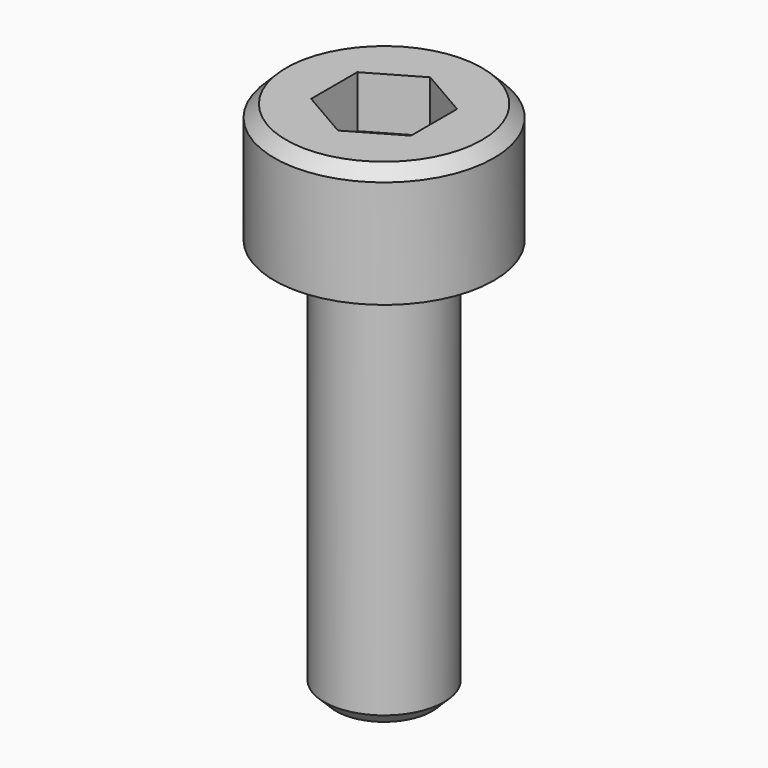
from build123d import *

# Parameters (mm, degrees)
F2_R      = 1.5
F3_DEPTH  = 10
F2_R_2    = 2.75
F3_FACE_R = 1.5
F4_DEPTH  = 3
F5_SIZE   = 0.3
F7_DEPTH  = 1.3


with BuildPart() as f3:
    # F2 (on Top) → F3 (new body)
    with BuildSketch(Plane.XY):
        Circle(F2_R)
    extrude(amount=-F3_DEPTH)

    # F2 (on Top) + F3_face (on face) → F4 (join)
    with BuildSketch(Plane.XY):
        Circle(F2_R_2)
        Circle(F2_R, mode=Mode.SUBTRACT)
    with BuildSketch(Plane.XY):
        Circle(F3_FACE_R)
    extrude(amount=F4_DEPTH)

    # F5
    f5_edges = [f3.edges().sort_by_distance(p)[0] for p in [
        (-1.5, 0, -10),
        (-2.75, 0, 3),
    ]]
    chamfer(f5_edges, length=F5_SIZE)

    # F6 (on face) → F7 (cut)
    with BuildSketch(Plane.XY.offset(3)):
        Polygon((1.25, -0.7216878365), (1.25, 0.7216878365), (0, 1.443375673), (-1.25, 0.7216878365), (-1.25, -0.7216878365), (0, -1.443375673), align=None)
    extrude(amount=-F7_DEPTH, mode=Mode.SUBTRACT)


solid = f3.part
